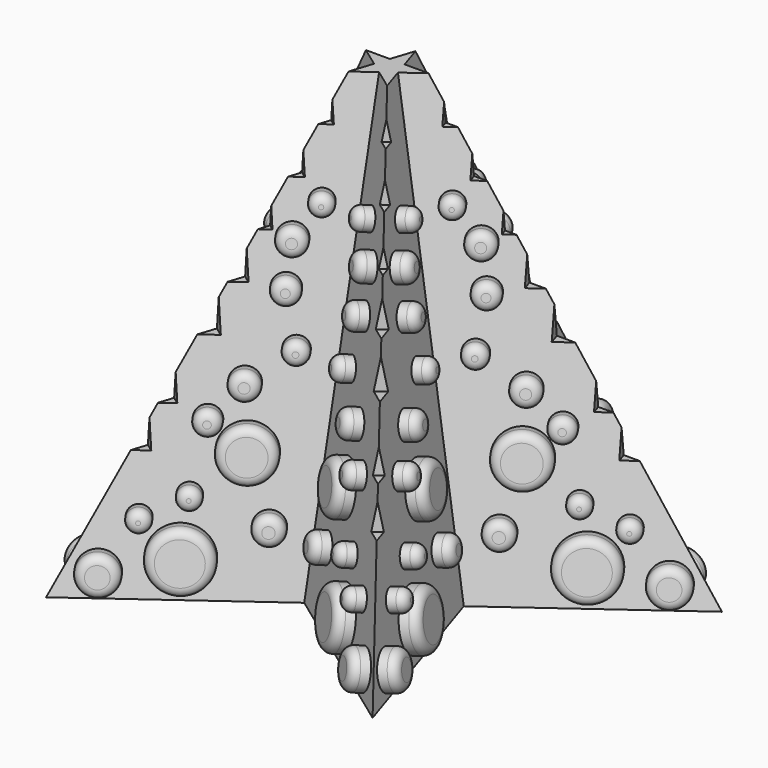
from build123d import *

# Parameters (mm, degrees)
F1_DEPTH               = 127
DRAFT_F1_DRAFTED_ANGLE = 10
F2_R                   = 17.4687003863
F2_R_2                 = 13.5858780078
F3_DEPTH               = 12.7
F2_R_3                 = 24.3755541597
F2_R_4                 = 20.5442302146
F4_DEPTH               = 25.4
F2_R_5                 = 34.1119304295
F2_R_6                 = 28.2437550543
F5_DEPTH               = 38.1
F2_R_7                 = 40.8197179688
F6_DEPTH               = 50.8
F2_R_8                 = 46.2786956803
F7_DEPTH               = 63.5
F2_R_9                 = 57.4118245149
F2_R_10                = 51.1444828457
F8_DEPTH               = 80.01
F2_R_11                = 65.4907810886
F9_DEPTH               = 91.44
F10_R                  = 3.1576728994
F11_DEPTH              = 5.08
F10_R_2                = 3.6989945995
F10_R_3                = 3.9374666193
F10_R_4                = 3.5428767899
F10_R_5                = 3.9500199555
F10_R_6                = 3.3324647961
F10_R_7                = 7.4930896274
F10_R_8                = 3.1326608725
F10_R_9                = 8.4309343855
F10_R_10               = 5.5044098198
F10_R_11               = 4.0915886639
F10_R_12               = 3.1153350046
F12_R                  = 2.54
F12_2_R                = 2.54
F12_3_R                = 2.54
F12_4_R                = 2.54
F12_5_R                = 2.54
F12_6_R                = 2.54
F12_7_R                = 2.54
F12_8_R                = 2.54
F12_9_R                = 2.54
F12_10_R               = 2.54
F12_11_R               = 2.54
F12_12_R               = 2.54
F13_COUNT              = 5
F15_COUNT              = 5
F16_R                  = 5.0597313891
F17_DEPTH              = 25.4


# Not quite as in the source:
# - an extrude with a draft is written as a straight extrude whose walls are then drafted


with BuildPart() as f1:
    # F0 (on Top) → F1 (new body)
    with BuildSketch(Plane.XY):
        Polygon((-18.4541802113, 25.4), (-78.1731618443, 25.4), (-29.8594908165, -9.7019366858), align=None)
        Polygon((-18.4541802113, 25.4), (-29.8594908165, -9.7019366858), (0, -31.3961266285), (29.8594908165, -9.7019366858), (18.4541802113, 25.4), align=None)
        Polygon((0, -31.3961266285), (-29.8594908165, -9.7019366858), (-48.3136710278, -66.4980633142), align=None)
        Polygon((0, 82.1961266285), (-18.4541802113, 25.4), (18.4541802113, 25.4), align=None)
        Polygon((29.8594908165, -9.7019366858), (0, -31.3961266285), (48.3136710278, -66.4980633142), align=None)
        Polygon((78.1731618443, 25.4), (18.4541802113, 25.4), (29.8594908165, -9.7019366858), align=None)
    extrude(amount=F1_DEPTH)

    # draft_F1_drafted
    draft_f1_drafted_walls = [f1.faces().sort_by_distance(p)[0] for p in [
        (-54.0163263304, 7.8490316571, 84.6666666667),
        (-39.0865809221, -38.1, 84.6666666667),
        (-24.1568355139, -48.9470949714, 84.6666666667),
        (24.1568355139, -48.9470949714, 84.6666666667),
        (39.0865809221, -38.1, 84.6666666667),
        (54.0163263304, 7.8490316571, 84.6666666667),
        (48.3136710278, 25.4, 84.6666666667),
        (9.2270901057, 53.7980633142, 84.6666666667),
        (-9.2270901057, 53.7980633142, 84.6666666667),
        (-48.3136710278, 25.4, 84.6666666667),
    ]]
    draft(draft_f1_drafted_walls, neutral_plane=Plane.XY, angle=DRAFT_F1_DRAFTED_ANGLE)

    # F2 (on face) → F3 (cut)
    with BuildSketch(Plane.XY.offset(127)):
        Circle(F2_R)
        Circle(F2_R_2, mode=Mode.SUBTRACT)
    extrude(amount=-F3_DEPTH, mode=Mode.SUBTRACT)

    # F2 (on face) → F4 (cut)
    with BuildSketch(Plane.XY.offset(127)):
        Circle(F2_R_3)
        Circle(F2_R_4, mode=Mode.SUBTRACT)
    extrude(amount=-F4_DEPTH, mode=Mode.SUBTRACT)

    # F2 (on face) → F5 (cut)
    with BuildSketch(Plane.XY.offset(127)):
        Circle(F2_R_5)
        Circle(F2_R_6, mode=Mode.SUBTRACT)
    extrude(amount=-F5_DEPTH, mode=Mode.SUBTRACT)

    # F2 (on face) → F6 (cut)
    with BuildSketch(Plane.XY.offset(127)):
        Circle(F2_R_7)
        Circle(F2_R_5, mode=Mode.SUBTRACT)
    extrude(amount=-F6_DEPTH, mode=Mode.SUBTRACT)

    # F2 (on face) → F7 (cut)
    with BuildSketch(Plane.XY.offset(127)):
        Circle(F2_R_8)
        Circle(F2_R_7, mode=Mode.SUBTRACT)
    extrude(amount=-F7_DEPTH, mode=Mode.SUBTRACT)

    # F2 (on face) → F8 (cut)
    with BuildSketch(Plane.XY.offset(127)):
        Circle(F2_R_9)
        Circle(F2_R_10, mode=Mode.SUBTRACT)
    extrude(amount=-F8_DEPTH, mode=Mode.SUBTRACT)

    # F2 (on face) → F9 (cut)
    with BuildSketch(Plane.XY.offset(127)):
        Circle(F2_R_11)
        Circle(F2_R_9, mode=Mode.SUBTRACT)
    extrude(amount=-F9_DEPTH, mode=Mode.SUBTRACT)


with BuildPart() as f11:
    # F10 (on face) → F11 (new body)
    with BuildSketch(Plane(origin=(-14.4795584993, -19.9294025348, 4.3436558202), x_dir=(0.8154301569, -0.5655779625, 0.1232689241), z_dir=(-0.5788554736, -0.7967262084, 0.1736481777))):
        with Locations((26.6408547759, 90.4996022582)):
            Circle(F10_R)
    extrude(amount=F11_DEPTH)

    # F12
    f12_edges = [f11.edges().sort_by_distance(p)[0] for p in [
        (1.72875, -17.986193, 96.544301),
    ]]
    fillet(f12_edges, radius=F12_R)


with BuildPart() as f11b:
    # F10 (on face) → F11, piece 2 (new body)
    with BuildSketch(Plane(origin=(-14.4795584993, -19.9294025348, 4.3436558202), x_dir=(0.8154301569, -0.5655779625, 0.1232689241), z_dir=(-0.5788554736, -0.7967262084, 0.1736481777))):
        with Locations((32.0492759347, 68.5065612197)):
            Circle(F10_R_2)
    extrude(amount=F11_DEPTH)

    # F12#2
    f12_2_edges = [f11b.edges().sort_by_distance(p)[0] for p in [
        (5.69753, -25.422398, 75.655688),
    ]]
    fillet(f12_2_edges, radius=F12_2_R)


with BuildPart() as f11c:
    # F10 (on face) → F11, piece 3 (new body)
    with BuildSketch(Plane(origin=(-14.4795584993, -19.9294025348, 4.3436558202), x_dir=(0.8154301569, -0.5655779625, 0.1232689241), z_dir=(-0.5788554736, -0.7967262084, 0.1736481777))):
        with Locations((32.2312638164, 80.6611403823)):
            Circle(F10_R_3)
    extrude(amount=F11_DEPTH)

    # F12#3
    f12_3_edges = [f11c.edges().sort_by_distance(p)[0] for p in [
        (5.651471, -22.8021, 87.524508),
    ]]
    fillet(f12_3_edges, radius=F12_3_R)


with BuildPart() as f11d:
    # F10 (on face) → F11, piece 4 (new body)
    with BuildSketch(Plane(origin=(-14.4795584993, -19.9294025348, 4.3436558202), x_dir=(0.8154301569, -0.5655779625, 0.1232689241), z_dir=(-0.5788554736, -0.7967262084, 0.1736481777))):
        with Locations((45.7290709019, 34.3072414398)):
            Circle(F10_R_4)
    extrude(amount=F11_DEPTH)

    # F12#4
    f12_4_edges = [f11d.edges().sort_by_distance(p)[0] for p in [
        (16.979751, -40.530528, 43.946354),
    ]]
    fillet(f12_4_edges, radius=F12_4_R)


with BuildPart() as f11e:
    # F10 (on face) → F11, piece 5 (new body)
    with BuildSketch(Plane(origin=(-14.4795584993, -19.9294025348, 4.3436558202), x_dir=(0.8154301569, -0.5655779625, 0.1232689241), z_dir=(-0.5788554736, -0.7967262084, 0.1736481777))):
        with Locations((38.4275242686, 44.3591747654)):
            Circle(F10_R_5)
    extrude(amount=F11_DEPTH)

    # F12#5
    f12_5_edges = [f11e.edges().sort_by_distance(p)[0] for p in [
        (10.693852, -34.030076, 52.817479),
    ]]
    fillet(f12_5_edges, radius=F12_5_R)


with BuildPart() as f11f:
    # F10 (on face) → F11, piece 6 (new body)
    with BuildSketch(Plane(origin=(-14.4795584993, -19.9294025348, 4.3436558202), x_dir=(0.8154301569, -0.5655779625, 0.1232689241), z_dir=(-0.5788554736, -0.7967262084, 0.1736481777))):
        with Locations((27.7298726141, 54.1249098866)):
            Circle(F10_R_6)
    extrude(amount=F11_DEPTH)

    # F12#6
    f12_6_edges = [f11f.edges().sort_by_distance(p)[0] for p in [
        (2.474238, -26.249354, 61.116649),
    ]]
    fillet(f12_6_edges, radius=F12_6_R)


with BuildPart() as f11g:
    # F10 (on face) → F11, piece 7 (new body)
    with BuildSketch(Plane(origin=(-14.4795584993, -19.9294025348, 4.3436558202), x_dir=(0.8154301569, -0.5655779625, 0.1232689241), z_dir=(-0.5788554736, -0.7967262084, 0.1736481777))):
        with Locations((35.5884246528, 27.8065185994)):
            Circle(F10_R_7)
    extrude(amount=F11_DEPTH)

    # F12#7
    f12_7_edges = [f11g.edges().sort_by_distance(p)[0] for p in [
        (5.489639, -33.945397, 35.857776),
    ]]
    fillet(f12_7_edges, radius=F12_7_R)


with BuildPart() as f11h:
    # F10 (on face) → F11, piece 8 (new body)
    with BuildSketch(Plane(origin=(-14.4795584993, -19.9294025348, 4.3436558202), x_dir=(0.8154301569, -0.5655779625, 0.1232689241), z_dir=(-0.5788554736, -0.7967262084, 0.1736481777))):
        with Locations((58.3128668368, 8.3645572886)):
            Circle(F10_R_8)
    extrude(amount=F11_DEPTH)

    # F12#8
    f12_8_edges = [f11h.edges().sort_by_distance(p)[0] for p in [
        (27.57546, -53.404224, 20.200488),
    ]]
    fillet(f12_8_edges, radius=F12_8_R)


with BuildPart() as f11i:
    # F10 (on face) → F11, piece 9 (new body)
    with BuildSketch(Plane(origin=(-14.4795584993, -19.9294025348, 4.3436558202), x_dir=(0.8154301569, -0.5655779625, 0.1232689241), z_dir=(-0.5788554736, -0.7967262084, 0.1736481777))):
        with Locations((47.4570728838, 0)):
            Circle(F10_R_9)
    extrude(amount=F11_DEPTH)

    # F12#9
    f12_9_edges = [f11i.edges().sort_by_distance(p)[0] for p in [
        (14.402946, -46.049096, 10.036499),
    ]]
    fillet(f12_9_edges, radius=F12_9_R)


with BuildPart() as f11j:
    # F10 (on face) → F11, piece 10 (new body)
    with BuildSketch(Plane(origin=(-14.4795584993, -19.9294025348, 4.3436558202), x_dir=(0.8154301569, -0.5655779625, 0.1232689241), z_dir=(-0.5788554736, -0.7967262084, 0.1736481777))):
        with Locations((65.894074738, -6.1225085519)):
            Circle(F10_R_10)
    extrude(amount=F11_DEPTH)

    # F12#10
    f12_10_edges = [f11j.edges().sort_by_distance(p)[0] for p in [
        (31.82341, -59.435641, 6.687884),
    ]]
    fillet(f12_10_edges, radius=F12_10_R)


with BuildPart() as f11k:
    # F10 (on face) → F11, piece 11 (new body)
    with BuildSketch(Plane(origin=(-14.4795584993, -19.9294025348, 4.3436558202), x_dir=(0.8154301569, -0.5655779625, 0.1232689241), z_dir=(-0.5788554736, -0.7967262084, 0.1736481777))):
        with Locations((28.1775780022, 10.4751829058)):
            Circle(F10_R_11)
    extrude(amount=F11_DEPTH)

    # F12#11
    f12_11_edges = [f11k.edges().sort_by_distance(p)[0] for p in [
        (2.220298, -35.368556, 18.429751),
    ]]
    fillet(f12_11_edges, radius=F12_11_R)


with BuildPart() as f11l:
    # F10 (on face) → F11, piece 12 (new body)
    with BuildSketch(Plane(origin=(-14.4795584993, -19.9294025348, 4.3436558202), x_dir=(0.8154301569, -0.5655779625, 0.1232689241), z_dir=(-0.5788554736, -0.7967262084, 0.1736481777))):
        with Locations((47.4570728838, 15.4326958582)):
            Circle(F10_R_12)
    extrude(amount=F11_DEPTH)

    # F12#12
    f12_12_edges = [f11l.edges().sort_by_distance(p)[0] for p in [
        (18.737446, -45.769045, 25.770455),
    ]]
    fillet(f12_12_edges, radius=F12_12_R)


with BuildPart() as f13_1:
    # F13: instance of F11
    add(f11.part.rotate(Axis((0, 0, 127), (0, 0, 1)), 1 * 360 / F13_COUNT))


with BuildPart() as f13_2:
    # F13: instance of F11
    add(f11.part.rotate(Axis((0, 0, 127), (0, 0, 1)), 2 * 360 / F13_COUNT))


with BuildPart() as f13_3:
    # F13: instance of F11
    add(f11.part.rotate(Axis((0, 0, 127), (0, 0, 1)), 3 * 360 / F13_COUNT))


with BuildPart() as f13_4:
    # F13: instance of F11
    add(f11.part.rotate(Axis((0, 0, 127), (0, 0, 1)), 4 * 360 / F13_COUNT))


with BuildPart() as f13_5:
    # F13: instance of F11b
    add(f11b.part.rotate(Axis((0, 0, 127), (0, 0, 1)), 1 * 360 / F13_COUNT))


with BuildPart() as f13_6:
    # F13: instance of F11b
    add(f11b.part.rotate(Axis((0, 0, 127), (0, 0, 1)), 2 * 360 / F13_COUNT))


with BuildPart() as f13_7:
    # F13: instance of F11b
    add(f11b.part.rotate(Axis((0, 0, 127), (0, 0, 1)), 3 * 360 / F13_COUNT))


with BuildPart() as f13_8:
    # F13: instance of F11b
    add(f11b.part.rotate(Axis((0, 0, 127), (0, 0, 1)), 4 * 360 / F13_COUNT))


with BuildPart() as f13_9:
    # F13: instance of F11c
    add(f11c.part.rotate(Axis((0, 0, 127), (0, 0, 1)), 1 * 360 / F13_COUNT))


with BuildPart() as f13_10:
    # F13: instance of F11c
    add(f11c.part.rotate(Axis((0, 0, 127), (0, 0, 1)), 2 * 360 / F13_COUNT))


with BuildPart() as f13_11:
    # F13: instance of F11c
    add(f11c.part.rotate(Axis((0, 0, 127), (0, 0, 1)), 3 * 360 / F13_COUNT))


with BuildPart() as f13_12:
    # F13: instance of F11c
    add(f11c.part.rotate(Axis((0, 0, 127), (0, 0, 1)), 4 * 360 / F13_COUNT))


with BuildPart() as f13_13:
    # F13: instance of F11d
    add(f11d.part.rotate(Axis((0, 0, 127), (0, 0, 1)), 1 * 360 / F13_COUNT))


with BuildPart() as f13_14:
    # F13: instance of F11d
    add(f11d.part.rotate(Axis((0, 0, 127), (0, 0, 1)), 2 * 360 / F13_COUNT))


with BuildPart() as f13_15:
    # F13: instance of F11d
    add(f11d.part.rotate(Axis((0, 0, 127), (0, 0, 1)), 3 * 360 / F13_COUNT))


with BuildPart() as f13_16:
    # F13: instance of F11d
    add(f11d.part.rotate(Axis((0, 0, 127), (0, 0, 1)), 4 * 360 / F13_COUNT))


with BuildPart() as f13_17:
    # F13: instance of F11e
    add(f11e.part.rotate(Axis((0, 0, 127), (0, 0, 1)), 1 * 360 / F13_COUNT))


with BuildPart() as f13_18:
    # F13: instance of F11e
    add(f11e.part.rotate(Axis((0, 0, 127), (0, 0, 1)), 2 * 360 / F13_COUNT))


with BuildPart() as f13_19:
    # F13: instance of F11e
    add(f11e.part.rotate(Axis((0, 0, 127), (0, 0, 1)), 3 * 360 / F13_COUNT))


with BuildPart() as f13_20:
    # F13: instance of F11e
    add(f11e.part.rotate(Axis((0, 0, 127), (0, 0, 1)), 4 * 360 / F13_COUNT))


with BuildPart() as f13_21:
    # F13: instance of F11f
    add(f11f.part.rotate(Axis((0, 0, 127), (0, 0, 1)), 1 * 360 / F13_COUNT))


with BuildPart() as f13_22:
    # F13: instance of F11f
    add(f11f.part.rotate(Axis((0, 0, 127), (0, 0, 1)), 2 * 360 / F13_COUNT))


with BuildPart() as f13_23:
    # F13: instance of F11f
    add(f11f.part.rotate(Axis((0, 0, 127), (0, 0, 1)), 3 * 360 / F13_COUNT))


with BuildPart() as f13_24:
    # F13: instance of F11f
    add(f11f.part.rotate(Axis((0, 0, 127), (0, 0, 1)), 4 * 360 / F13_COUNT))


with BuildPart() as f13_25:
    # F13: instance of F11g
    add(f11g.part.rotate(Axis((0, 0, 127), (0, 0, 1)), 1 * 360 / F13_COUNT))


with BuildPart() as f13_26:
    # F13: instance of F11g
    add(f11g.part.rotate(Axis((0, 0, 127), (0, 0, 1)), 2 * 360 / F13_COUNT))


with BuildPart() as f13_27:
    # F13: instance of F11g
    add(f11g.part.rotate(Axis((0, 0, 127), (0, 0, 1)), 3 * 360 / F13_COUNT))


with BuildPart() as f13_28:
    # F13: instance of F11g
    add(f11g.part.rotate(Axis((0, 0, 127), (0, 0, 1)), 4 * 360 / F13_COUNT))


with BuildPart() as f13_29:
    # F13: instance of F11h
    add(f11h.part.rotate(Axis((0, 0, 127), (0, 0, 1)), 1 * 360 / F13_COUNT))


with BuildPart() as f13_30:
    # F13: instance of F11h
    add(f11h.part.rotate(Axis((0, 0, 127), (0, 0, 1)), 2 * 360 / F13_COUNT))


with BuildPart() as f13_31:
    # F13: instance of F11h
    add(f11h.part.rotate(Axis((0, 0, 127), (0, 0, 1)), 3 * 360 / F13_COUNT))


with BuildPart() as f13_32:
    # F13: instance of F11h
    add(f11h.part.rotate(Axis((0, 0, 127), (0, 0, 1)), 4 * 360 / F13_COUNT))


with BuildPart() as f13_33:
    # F13: instance of F11i
    add(f11i.part.rotate(Axis((0, 0, 127), (0, 0, 1)), 1 * 360 / F13_COUNT))


with BuildPart() as f13_34:
    # F13: instance of F11i
    add(f11i.part.rotate(Axis((0, 0, 127), (0, 0, 1)), 2 * 360 / F13_COUNT))


with BuildPart() as f13_35:
    # F13: instance of F11i
    add(f11i.part.rotate(Axis((0, 0, 127), (0, 0, 1)), 3 * 360 / F13_COUNT))


with BuildPart() as f13_36:
    # F13: instance of F11i
    add(f11i.part.rotate(Axis((0, 0, 127), (0, 0, 1)), 4 * 360 / F13_COUNT))


with BuildPart() as f13_37:
    # F13: instance of F11j
    add(f11j.part.rotate(Axis((0, 0, 127), (0, 0, 1)), 1 * 360 / F13_COUNT))


with BuildPart() as f13_38:
    # F13: instance of F11j
    add(f11j.part.rotate(Axis((0, 0, 127), (0, 0, 1)), 2 * 360 / F13_COUNT))


with BuildPart() as f13_39:
    # F13: instance of F11j
    add(f11j.part.rotate(Axis((0, 0, 127), (0, 0, 1)), 3 * 360 / F13_COUNT))


with BuildPart() as f13_40:
    # F13: instance of F11j
    add(f11j.part.rotate(Axis((0, 0, 127), (0, 0, 1)), 4 * 360 / F13_COUNT))


with BuildPart() as f13_41:
    # F13: instance of F11k
    add(f11k.part.rotate(Axis((0, 0, 127), (0, 0, 1)), 1 * 360 / F13_COUNT))


with BuildPart() as f13_42:
    # F13: instance of F11k
    add(f11k.part.rotate(Axis((0, 0, 127), (0, 0, 1)), 2 * 360 / F13_COUNT))


with BuildPart() as f13_43:
    # F13: instance of F11k
    add(f11k.part.rotate(Axis((0, 0, 127), (0, 0, 1)), 3 * 360 / F13_COUNT))


with BuildPart() as f13_44:
    # F13: instance of F11k
    add(f11k.part.rotate(Axis((0, 0, 127), (0, 0, 1)), 4 * 360 / F13_COUNT))


with BuildPart() as f13_45:
    # F13: instance of F11l
    add(f11l.part.rotate(Axis((0, 0, 127), (0, 0, 1)), 1 * 360 / F13_COUNT))


with BuildPart() as f13_46:
    # F13: instance of F11l
    add(f11l.part.rotate(Axis((0, 0, 127), (0, 0, 1)), 2 * 360 / F13_COUNT))


with BuildPart() as f13_47:
    # F13: instance of F11l
    add(f11l.part.rotate(Axis((0, 0, 127), (0, 0, 1)), 3 * 360 / F13_COUNT))


with BuildPart() as f13_48:
    # F13: instance of F11l
    add(f11l.part.rotate(Axis((0, 0, 127), (0, 0, 1)), 4 * 360 / F13_COUNT))


with BuildPart() as f14_1:
    # F14: instance of F13_2
    add(f13_2.part.mirror(Plane.YZ))


with BuildPart() as f14_2:
    # F14: instance of F13_10
    add(f13_10.part.mirror(Plane.YZ))


with BuildPart() as f14_3:
    # F14: instance of F13_6
    add(f13_6.part.mirror(Plane.YZ))


with BuildPart() as f14_4:
    # F14: instance of F13_22
    add(f13_22.part.mirror(Plane.YZ))


with BuildPart() as f14_5:
    # F14: instance of F13_18
    add(f13_18.part.mirror(Plane.YZ))


with BuildPart() as f14_6:
    # F14: instance of F13_14
    add(f13_14.part.mirror(Plane.YZ))


with BuildPart() as f14_7:
    # F14: instance of F13_26
    add(f13_26.part.mirror(Plane.YZ))


with BuildPart() as f14_8:
    # F14: instance of F13_42
    add(f13_42.part.mirror(Plane.YZ))


with BuildPart() as f14_9:
    # F14: instance of F13_46
    add(f13_46.part.mirror(Plane.YZ))


with BuildPart() as f14_10:
    # F14: instance of F13_30
    add(f13_30.part.mirror(Plane.YZ))


with BuildPart() as f14_11:
    # F14: instance of F13_38
    add(f13_38.part.mirror(Plane.YZ))


with BuildPart() as f14_12:
    # F14: instance of F13_34
    add(f13_34.part.mirror(Plane.YZ))


with BuildPart() as f15_1:
    # F15: instance of F14_1
    add(f14_1.part.rotate(Axis((0, 0, 127), (0, 0, 1)), 1 * 360 / F15_COUNT))


with BuildPart() as f15_2:
    # F15: instance of F14_1
    add(f14_1.part.rotate(Axis((0, 0, 127), (0, 0, 1)), 2 * 360 / F15_COUNT))


with BuildPart() as f15_3:
    # F15: instance of F14_1
    add(f14_1.part.rotate(Axis((0, 0, 127), (0, 0, 1)), 3 * 360 / F15_COUNT))


with BuildPart() as f15_4:
    # F15: instance of F14_1
    add(f14_1.part.rotate(Axis((0, 0, 127), (0, 0, 1)), 4 * 360 / F15_COUNT))


with BuildPart() as f15_5:
    # F15: instance of F14_2
    add(f14_2.part.rotate(Axis((0, 0, 127), (0, 0, 1)), 1 * 360 / F15_COUNT))


with BuildPart() as f15_6:
    # F15: instance of F14_2
    add(f14_2.part.rotate(Axis((0, 0, 127), (0, 0, 1)), 2 * 360 / F15_COUNT))


with BuildPart() as f15_7:
    # F15: instance of F14_2
    add(f14_2.part.rotate(Axis((0, 0, 127), (0, 0, 1)), 3 * 360 / F15_COUNT))


with BuildPart() as f15_8:
    # F15: instance of F14_2
    add(f14_2.part.rotate(Axis((0, 0, 127), (0, 0, 1)), 4 * 360 / F15_COUNT))


with BuildPart() as f15_9:
    # F15: instance of F14_3
    add(f14_3.part.rotate(Axis((0, 0, 127), (0, 0, 1)), 1 * 360 / F15_COUNT))


with BuildPart() as f15_10:
    # F15: instance of F14_3
    add(f14_3.part.rotate(Axis((0, 0, 127), (0, 0, 1)), 2 * 360 / F15_COUNT))


with BuildPart() as f15_11:
    # F15: instance of F14_3
    add(f14_3.part.rotate(Axis((0, 0, 127), (0, 0, 1)), 3 * 360 / F15_COUNT))


with BuildPart() as f15_12:
    # F15: instance of F14_3
    add(f14_3.part.rotate(Axis((0, 0, 127), (0, 0, 1)), 4 * 360 / F15_COUNT))


with BuildPart() as f15_13:
    # F15: instance of F14_4
    add(f14_4.part.rotate(Axis((0, 0, 127), (0, 0, 1)), 1 * 360 / F15_COUNT))


with BuildPart() as f15_14:
    # F15: instance of F14_4
    add(f14_4.part.rotate(Axis((0, 0, 127), (0, 0, 1)), 2 * 360 / F15_COUNT))


with BuildPart() as f15_15:
    # F15: instance of F14_4
    add(f14_4.part.rotate(Axis((0, 0, 127), (0, 0, 1)), 3 * 360 / F15_COUNT))


with BuildPart() as f15_16:
    # F15: instance of F14_4
    add(f14_4.part.rotate(Axis((0, 0, 127), (0, 0, 1)), 4 * 360 / F15_COUNT))


with BuildPart() as f15_17:
    # F15: instance of F14_7
    add(f14_7.part.rotate(Axis((0, 0, 127), (0, 0, 1)), 1 * 360 / F15_COUNT))


with BuildPart() as f15_18:
    # F15: instance of F14_7
    add(f14_7.part.rotate(Axis((0, 0, 127), (0, 0, 1)), 2 * 360 / F15_COUNT))


with BuildPart() as f15_19:
    # F15: instance of F14_7
    add(f14_7.part.rotate(Axis((0, 0, 127), (0, 0, 1)), 3 * 360 / F15_COUNT))


with BuildPart() as f15_20:
    # F15: instance of F14_7
    add(f14_7.part.rotate(Axis((0, 0, 127), (0, 0, 1)), 4 * 360 / F15_COUNT))


with BuildPart() as f15_21:
    # F15: instance of F14_5
    add(f14_5.part.rotate(Axis((0, 0, 127), (0, 0, 1)), 1 * 360 / F15_COUNT))


with BuildPart() as f15_22:
    # F15: instance of F14_5
    add(f14_5.part.rotate(Axis((0, 0, 127), (0, 0, 1)), 2 * 360 / F15_COUNT))


with BuildPart() as f15_23:
    # F15: instance of F14_5
    add(f14_5.part.rotate(Axis((0, 0, 127), (0, 0, 1)), 3 * 360 / F15_COUNT))


with BuildPart() as f15_24:
    # F15: instance of F14_5
    add(f14_5.part.rotate(Axis((0, 0, 127), (0, 0, 1)), 4 * 360 / F15_COUNT))


with BuildPart() as f15_25:
    # F15: instance of F14_6
    add(f14_6.part.rotate(Axis((0, 0, 127), (0, 0, 1)), 1 * 360 / F15_COUNT))


with BuildPart() as f15_26:
    # F15: instance of F14_6
    add(f14_6.part.rotate(Axis((0, 0, 127), (0, 0, 1)), 2 * 360 / F15_COUNT))


with BuildPart() as f15_27:
    # F15: instance of F14_6
    add(f14_6.part.rotate(Axis((0, 0, 127), (0, 0, 1)), 3 * 360 / F15_COUNT))


with BuildPart() as f15_28:
    # F15: instance of F14_6
    add(f14_6.part.rotate(Axis((0, 0, 127), (0, 0, 1)), 4 * 360 / F15_COUNT))


with BuildPart() as f15_29:
    # F15: instance of F14_9
    add(f14_9.part.rotate(Axis((0, 0, 127), (0, 0, 1)), 1 * 360 / F15_COUNT))


with BuildPart() as f15_30:
    # F15: instance of F14_9
    add(f14_9.part.rotate(Axis((0, 0, 127), (0, 0, 1)), 2 * 360 / F15_COUNT))


with BuildPart() as f15_31:
    # F15: instance of F14_9
    add(f14_9.part.rotate(Axis((0, 0, 127), (0, 0, 1)), 3 * 360 / F15_COUNT))


with BuildPart() as f15_32:
    # F15: instance of F14_9
    add(f14_9.part.rotate(Axis((0, 0, 127), (0, 0, 1)), 4 * 360 / F15_COUNT))


with BuildPart() as f15_33:
    # F15: instance of F14_8
    add(f14_8.part.rotate(Axis((0, 0, 127), (0, 0, 1)), 1 * 360 / F15_COUNT))


with BuildPart() as f15_34:
    # F15: instance of F14_8
    add(f14_8.part.rotate(Axis((0, 0, 127), (0, 0, 1)), 2 * 360 / F15_COUNT))


with BuildPart() as f15_35:
    # F15: instance of F14_8
    add(f14_8.part.rotate(Axis((0, 0, 127), (0, 0, 1)), 3 * 360 / F15_COUNT))


with BuildPart() as f15_36:
    # F15: instance of F14_8
    add(f14_8.part.rotate(Axis((0, 0, 127), (0, 0, 1)), 4 * 360 / F15_COUNT))


with BuildPart() as f15_37:
    # F15: instance of F14_12
    add(f14_12.part.rotate(Axis((0, 0, 127), (0, 0, 1)), 1 * 360 / F15_COUNT))


with BuildPart() as f15_38:
    # F15: instance of F14_12
    add(f14_12.part.rotate(Axis((0, 0, 127), (0, 0, 1)), 2 * 360 / F15_COUNT))


with BuildPart() as f15_39:
    # F15: instance of F14_12
    add(f14_12.part.rotate(Axis((0, 0, 127), (0, 0, 1)), 3 * 360 / F15_COUNT))


with BuildPart() as f15_40:
    # F15: instance of F14_12
    add(f14_12.part.rotate(Axis((0, 0, 127), (0, 0, 1)), 4 * 360 / F15_COUNT))


with BuildPart() as f15_41:
    # F15: instance of F14_10
    add(f14_10.part.rotate(Axis((0, 0, 127), (0, 0, 1)), 1 * 360 / F15_COUNT))


with BuildPart() as f15_42:
    # F15: instance of F14_10
    add(f14_10.part.rotate(Axis((0, 0, 127), (0, 0, 1)), 2 * 360 / F15_COUNT))


with BuildPart() as f15_43:
    # F15: instance of F14_10
    add(f14_10.part.rotate(Axis((0, 0, 127), (0, 0, 1)), 3 * 360 / F15_COUNT))


with BuildPart() as f15_44:
    # F15: instance of F14_10
    add(f14_10.part.rotate(Axis((0, 0, 127), (0, 0, 1)), 4 * 360 / F15_COUNT))


with BuildPart() as f15_45:
    # F15: instance of F14_11
    add(f14_11.part.rotate(Axis((0, 0, 127), (0, 0, 1)), 1 * 360 / F15_COUNT))


with BuildPart() as f15_46:
    # F15: instance of F14_11
    add(f14_11.part.rotate(Axis((0, 0, 127), (0, 0, 1)), 2 * 360 / F15_COUNT))


with BuildPart() as f15_47:
    # F15: instance of F14_11
    add(f14_11.part.rotate(Axis((0, 0, 127), (0, 0, 1)), 3 * 360 / F15_COUNT))


with BuildPart() as f15_48:
    # F15: instance of F14_11
    add(f14_11.part.rotate(Axis((0, 0, 127), (0, 0, 1)), 4 * 360 / F15_COUNT))


with BuildPart() as f17:
    # F16 (on face) → F17 (new body)
    with BuildSketch(Plane(origin=(0, 0, 0), x_dir=(1, 0, 0), z_dir=(0, 0, -1))):
        Circle(F16_R)
    extrude(amount=F17_DEPTH)


solid = Compound([f1.part, f11.part, f11b.part, f11c.part, f11d.part, f11e.part, f11f.part, f11g.part, f11h.part, f11i.part, f11j.part, f11k.part, f11l.part, f13_1.part, f13_2.part, f13_3.part, f13_4.part, f13_5.part, f13_6.part, f13_7.part, f13_8.part, f13_9.part, f13_10.part, f13_11.part, f13_12.part, f13_13.part, f13_14.part, f13_15.part, f13_16.part, f13_17.part, f13_18.part, f13_19.part, f13_20.part, f13_21.part, f13_22.part, f13_23.part, f13_24.part, f13_25.part, f13_26.part, f13_27.part, f13_28.part, f13_29.part, f13_30.part, f13_31.part, f13_32.part, f13_33.part, f13_34.part, f13_35.part, f13_36.part, f13_37.part, f13_38.part, f13_39.part, f13_40.part, f13_41.part, f13_42.part, f13_43.part, f13_44.part, f13_45.part, f13_46.part, f13_47.part, f13_48.part, f14_1.part, f14_2.part, f14_3.part, f14_4.part, f14_5.part, f14_6.part, f14_7.part, f14_8.part, f14_9.part, f14_10.part, f14_11.part, f14_12.part, f15_1.part, f15_2.part, f15_3.part, f15_4.part, f15_5.part, f15_6.part, f15_7.part, f15_8.part, f15_9.part, f15_10.part, f15_11.part, f15_12.part, f15_13.part, f15_14.part, f15_15.part, f15_16.part, f15_17.part, f15_18.part, f15_19.part, f15_20.part, f15_21.part, f15_22.part, f15_23.part, f15_24.part, f15_25.part, f15_26.part, f15_27.part, f15_28.part, f15_29.part, f15_30.part, f15_31.part, f15_32.part, f15_33.part, f15_34.part, f15_35.part, f15_36.part, f15_37.part, f15_38.part, f15_39.part, f15_40.part, f15_41.part, f15_42.part, f15_43.part, f15_44.part, f15_45.part, f15_46.part, f15_47.part, f15_48.part, f17.part])
